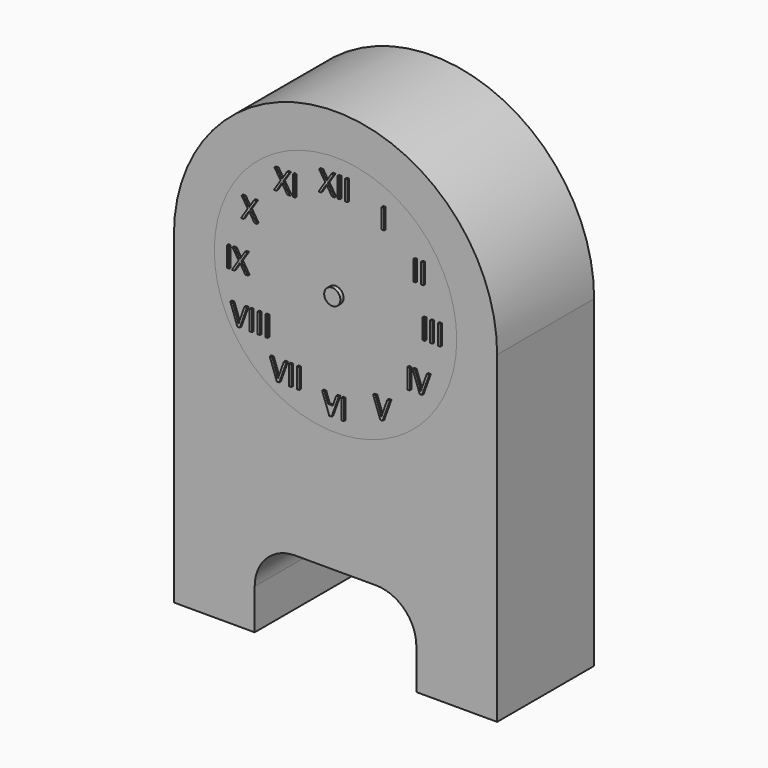
from build123d import *

# Parameters (mm, degrees)
F0_R         = 30
F1_DEPTH     = 30
F2_R         = 30
F3_DEPTH     = 10
F4_W         = 0.576171875
F4_H         = 2.4576822917
F4_H_2       = 2.5
F4_TEXT_SIZE = 6.9444444444
F5_DEPTH     = 0.5
F6_R         = 2
F7_DEPTH     = 1


# Not quite as in the source:
# - Text() gives the source's letters only with a copy of the font that has no kerning and outlines rounded to 1/6400 em; it was checked with that copy


with BuildPart() as f1:
    # F0 (on Front) → F1 (new body)
    with BuildSketch(Plane.XZ):
        with BuildLine():
            ThreePointArc((40, 0), (0, 40), (-40, 0))
            Line((-40, 0), (-40, -80))
            Line((-40, -80), (-20, -80))
            Line((-20, -80), (-20, -70))
            ThreePointArc((-20, -70), (-17.0710678119, -62.9289321881), (-10, -60))
            Line((-10, -60), (10, -60))
            ThreePointArc((10, -60), (17.0710678119, -62.9289321881), (20, -70))
            Line((20, -70), (20, -80))
            Line((20, -80), (40, -80))
            Line((40, -80), (40, 0))
        make_face()
        Circle(F0_R, mode=Mode.SUBTRACT)
    extrude(amount=F1_DEPTH)


with BuildPart() as f3:
    # F2 (on face) → F3 (new body)
    with BuildSketch(Plane.XZ.offset(30)):
        Circle(F2_R)
    extrude(amount=-F3_DEPTH)

    # F4 (on face) → F5 (join)
    with BuildSketch(Plane.XZ.offset(30)):
        Polygon((-2.9204644097, -21.5423177083), (-2.0393780465, -24), (-1.4365776176, -24), (-2.3095703125, -21.5423177083), align=None)
        with BuildLine():
            Line((-1.4365776176, -24), (-2.0393780465, -24))
            Line((-2.0393780465, -24), (-1.1431206597, -26.5))
            Line((-1.1431206597, -26.5), (-0.5734592014, -26.5))
            Line((-0.5734592014, -26.5), (0.3271755108, -24))
            Line((0.3271755108, -24), (-0.2803316427, -24))
            Line((-0.2803316427, -24), (-0.5398220486, -24.7302517361))
            add(Edge.make_bspline(
                [(-0.8588324653, -25.8250868056), (-0.7362196181, -25.2760416667), (-0.5398220486, -24.7302517361)],
                knots=[0, 0, 0, 1, 1, 1], degree=2))
            add(Edge.make_bspline(
                [(-1.1702473958, -24.7497829861), (-0.9738498264, -25.3031684028), (-0.8588324653, -25.8250868056)],
                knots=[0, 0, 0, 1, 1, 1], degree=2))
            Line((-1.1702473958, -24.7497829861), (-1.4365776176, -24))
        make_face()
        with Locations((2.1820746528, -22.7711588542)):
            Rectangle(F4_W, F4_H)
        with Locations((2.1820746528, -25.25)):
            Rectangle(F4_W, F4_H_2)
        with BuildLine():
            Line((-0.2803316427, -24), (-1.4365776176, -24))
            Line((-1.4365776176, -24), (-1.1702473958, -24.7497829861))
            add(Edge.make_bspline(
                [(-1.1702473958, -24.7497829861), (-0.9738498264, -25.3031684028), (-0.8588324653, -25.8250868056)],
                knots=[0, 0, 0, 1, 1, 1], degree=2))
            add(Edge.make_bspline(
                [(-0.8588324653, -25.8250868056), (-0.7362196181, -25.2760416667), (-0.5398220486, -24.7302517361)],
                knots=[0, 0, 0, 1, 1, 1], degree=2))
            Line((-0.5398220486, -24.7302517361), (-0.2803316427, -24))
        make_face()
        Polygon((0.5929904514, -21.5423177083), (-0.2803316427, -24), (0.3271755108, -24), (1.2125651042, -21.5423177083), align=None)
        with Locations((-3.8259548611, 21.5)):
            Text('XII', F4_TEXT_SIZE, font='Open Sans', text_align=(TextAlign.LEFT, TextAlign.BOTTOM))
        with Locations((11.1460503472, 18.2846096908)):
            Text('I', F4_TEXT_SIZE, font='Open Sans', text_align=(TextAlign.LEFT, TextAlign.BOTTOM))
        with Locations((18.9627780936, 9.5)):
            Text('II', F4_TEXT_SIZE, font='Open Sans', text_align=(TextAlign.LEFT, TextAlign.BOTTOM))
        with Locations((21.2102864583, -2.5)):
            Text('III', F4_TEXT_SIZE, font='Open Sans', text_align=(TextAlign.LEFT, TextAlign.BOTTOM))
        with Locations((17.5250610797, -14.5)):
            Text('IV', F4_TEXT_SIZE, font='Open Sans', text_align=(TextAlign.LEFT, TextAlign.BOTTOM))
        with Locations((9.7083333333, -23.2846096908)):
            Text('V', F4_TEXT_SIZE, font='Open Sans', text_align=(TextAlign.LEFT, TextAlign.BOTTOM))
        with Locations((-15.8883463542, -23.2846096908)):
            Text('VII', F4_TEXT_SIZE, font='Open Sans', text_align=(TextAlign.LEFT, TextAlign.BOTTOM))
        with Locations((-25.6408379894, -14.5)):
            Text('VIII', F4_TEXT_SIZE, font='Open Sans', text_align=(TextAlign.LEFT, TextAlign.BOTTOM))
        with Locations((-27.18359375, -2.5)):
            Text('IX', F4_TEXT_SIZE, font='Open Sans', text_align=(TextAlign.LEFT, TextAlign.BOTTOM))
        with Locations((-23.0003214964, 9.5)):
            Text('X', F4_TEXT_SIZE, font='Open Sans', text_align=(TextAlign.LEFT, TextAlign.BOTTOM))
        with Locations((-14.8580729167, 18.2846096908)):
            Text('XI', F4_TEXT_SIZE, font='Open Sans', text_align=(TextAlign.LEFT, TextAlign.BOTTOM))
    extrude(amount=F5_DEPTH)


with BuildPart() as f7:
    # F6 (on face) → F7 (new body)
    with BuildSketch(Plane.XZ.offset(30)):
        Circle(F6_R)
    extrude(amount=F7_DEPTH)


solid = Compound([f1.part, f3.part, f7.part])
